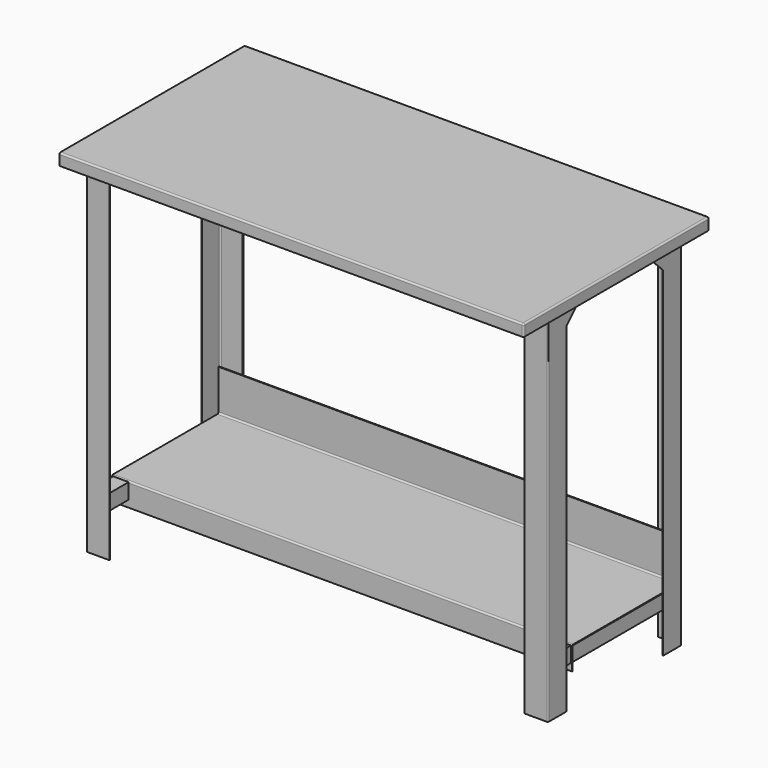
from build123d import *

# Parameters (mm, degrees)
F0_W          = 1524
F0_H          = 762
F1_DEPTH      = 2.65684
F2_W          = 2.65684
F2_H          = 2.65684
F2_W_2        = 1518.68632
F2_H_2        = 756.68632
F3_DEPTH      = 38.1
F4_R          = 5.31368
F6_DEPTH      = 1193.8
F7_R          = 3.98526
F8_R          = 3.98526
F9_W          = 50.8
F9_H          = 50.8
F10_DEPTH     = 542.85896
F12_DEPTH     = 1508.05896
F13_T1_DEPTH  = 1423.88844
F13_T6_DEPTH  = 1533.45896
F13_T9_DEPTH  = 1398.48844
F13_T14_DEPTH = 1533.45896
F13_T19_DEPTH = 1533.45896
F13_T24_DEPTH = 1533.45896
F13_T30_DEPTH = 1533.45896
F15_DEPTH     = 2.65684
F17_DEPTH     = 2.65684
F19_DEPTH     = 2.65684


# Not quite as in the source:
# - a fillet or chamfer that OpenCascade refuses, or shapes differently, is made with other operations: its cross-section is extruded or revolved along the edge and cut away or added
# - a pattern or mirror of a feature is missing from the dataset's text; its kind, count and spacing are read off the source's solid


with BuildPart() as f1:
    # F0 (on Top) → F1 (new body)
    with BuildSketch(Plane.XY):
        Rectangle(F0_W, F0_H)
    extrude(amount=F1_DEPTH)

    # F2 (on face) → F3 (join)
    with BuildSketch(Plane.XY.offset(2.65684)):
        with Locations((-760.67158, -379.67158)):
            Rectangle(F2_W, F2_H)
        with Locations((0, -379.67158)):
            Rectangle(F2_W_2, F2_H)
        with Locations((-760.67158, 0)):
            Rectangle(F2_W, F2_H_2)
        with Locations((760.67158, -379.67158)):
            Rectangle(F2_W, F2_H)
        with Locations((-760.67158, 379.67158)):
            Rectangle(F2_W, F2_H)
        with Locations((760.67158, 0)):
            Rectangle(F2_W, F2_H_2)
        with Locations((0, 379.67158)):
            Rectangle(F2_W_2, F2_H)
        with Locations((760.67158, 379.67158)):
            Rectangle(F2_W, F2_H)
    extrude(amount=-F3_DEPTH)

    # F4
    f4_edges = [f1.edges().sort_by_distance(p)[0] for p in [
        (-762, -381, -16.39316),
        (762, -381, -16.39316),
        (762, 381, -16.39316),
        (-762, 381, -16.39316),
        (-762, 0, 2.65684),
        (0, 381, 2.65684),
        (0, -381, 2.65684),
        (762, 0, 2.65684),
    ]]
    fillet(f4_edges, radius=F4_R)

    # F5 (on face) → F6 (join)
    with BuildSketch(Plane.XY.offset(2.65684)):
        Polygon((-680.48632, 274.08632), (-756.68632, 274.08632), (-756.68632, 197.88632), (-754.02948, 197.88632), (-754.02948, 271.42948), (-680.48632, 271.42948), align=None)
        Polygon((754.02948, 197.88632), (756.68632, 197.88632), (756.68632, 274.08632), (680.48632, 274.08632), (680.48632, 271.42948), (754.02948, 271.42948), align=None)
        Polygon((680.48632, -271.42948), (680.48632, -274.08632), (756.68632, -274.08632), (756.68632, -197.88632), (754.02948, -197.88632), (754.02948, -271.42948), align=None)
        Polygon((-754.02948, -197.88632), (-756.68632, -197.88632), (-756.68632, -274.08632), (-680.48632, -274.08632), (-680.48632, -271.42948), (-754.02948, -271.42948), align=None)
    extrude(amount=-F6_DEPTH)

    # F7
    f7_edges = [f1.edges().sort_by_distance(p)[0] for p in [
        (756.68632, 274.08632, -595.57158),
        (-756.68632, 274.08632, -595.57158),
        (-756.68632, -274.08632, -595.57158),
        (756.68632, -274.08632, -595.57158),
    ]]
    fillet(f7_edges, radius=F7_R)

    # F8
    f8_edges = [f1.edges().sort_by_distance(p)[0] for p in [
        (-754.02948, -271.42948, -595.57158),
        (-754.02948, 271.42948, -595.57158),
        (754.02948, -271.42948, -595.57158),
        (754.02948, 271.42948, -595.57158),
    ]]
    fillet(f8_edges, radius=F8_R)

    # F9 (on face) → F10 (join, through all)
    with BuildSketch(Plane(origin=(0, -271.42948, 0), x_dir=(-1, 0, 0), z_dir=(0, 1, 0))):
        with Locations((724.64422, -1038.74316)):
            Rectangle(F9_W, F9_H)
        with Locations((-724.64422, -1038.74316)):
            Rectangle(F9_W, F9_H)
    extrude(amount=F10_DEPTH)

    # F11 (on face) → F12 (join, through all)
    with BuildSketch(Plane(origin=(754.02948, 0, 0), x_dir=(0, -1, 0), z_dir=(-1, 0, 0))):
        Polygon((-267.44422, -876.0097688131), (-267.44422, -1013.34316), (169.82948, -1013.34316), (169.82948, -1086.88632), (172.48632, -1086.88632), (172.48632, -1010.68632), (-264.78738, -1010.68632), (-264.78738, -876.0097688131), align=None)
    extrude(amount=F12_DEPTH)

    # F13: fillet of radius 5.08 on 4 edges, made by hand

    # F13_s2 → F13_t1 (join)
    with BuildSketch(Plane.YZ.offset(-711.94422)):
        with BuildLine():
            ThreePointArc((-169.82948, -1018.42316), (-168.3415824484, -1014.8310575516), (-164.74948, -1013.34316))
            Line((-164.74948, -1013.34316), (-169.82948, -1013.34316))
            Line((-169.82948, -1013.34316), (-169.82948, -1018.42316))
        make_face()
    extrude(amount=F13_T1_DEPTH)


with BuildPart() as f13_tool4:
    # F13_s5 → F13_t6 (new body)
    with BuildSketch(Plane.YZ.offset(766.72948)):
        with BuildLine():
            ThreePointArc((264.78738, -1005.60632), (263.2994824484, -1009.1984224484), (259.70738, -1010.68632))
            Line((259.70738, -1010.68632), (264.78738, -1010.68632))
            Line((264.78738, -1010.68632), (264.78738, -1005.60632))
        make_face()
    extrude(amount=-F13_T6_DEPTH)

    split(bisect_by=Plane.YZ.offset(-756.68632), keep=Keep.TOP)

    split(bisect_by=Plane.YZ.offset(756.68632), keep=Keep.BOTTOM)


with BuildPart() as f1_1:
    add(f1.part)

    # F13_t3: union F13_tool4
    add(f13_tool4.part)

    # F13_s10 → F13_t9 (cut)
    with BuildSketch(Plane.YZ.offset(-699.24422)):
        with BuildLine():
            ThreePointArc((267.44422, -1008.26316), (265.9563224484, -1011.8552624484), (262.36422, -1013.34316))
            Line((262.36422, -1013.34316), (267.44422, -1013.34316))
            Line((267.44422, -1013.34316), (267.44422, -1008.26316))
        make_face()
    extrude(amount=F13_T9_DEPTH, mode=Mode.SUBTRACT)


with BuildPart() as f13_tool12:
    # F13_s13 → F13_t14 (new body)
    with BuildSketch(Plane.YZ.offset(766.72948)):
        with BuildLine():
            ThreePointArc((-167.40632, -1010.68632), (-170.9984224484, -1012.1742175516), (-172.48632, -1015.76632))
            Line((-172.48632, -1015.76632), (-172.48632, -1010.68632))
            Line((-172.48632, -1010.68632), (-167.40632, -1010.68632))
        make_face()
    extrude(amount=-F13_T14_DEPTH)

    split(bisect_by=Plane.XY.offset(-1013.34316), keep=Keep.TOP)


with BuildPart() as f1_2:
    add(f1_1.part)

    # F13_t11: cut F13_tool12
    add(f13_tool12.part, mode=Mode.SUBTRACT)


with BuildPart() as f13_tool17:
    # F13_s18 → F13_t19 (new body)
    with BuildSketch(Plane.YZ.offset(766.72948)):
        with BuildLine():
            ThreePointArc((-167.40632, -1010.68632), (-170.9984224484, -1012.1742175516), (-172.48632, -1015.76632))
            Line((-172.48632, -1015.76632), (-172.48632, -1010.68632))
            Line((-172.48632, -1010.68632), (-167.40632, -1010.68632))
        make_face()
    extrude(amount=-F13_T19_DEPTH)

    split(bisect_by=Plane.YZ.offset(750.04422), keep=Keep.TOP)


with BuildPart() as f1_3:
    add(f1_2.part)

    # F13_t16: cut F13_tool17
    add(f13_tool17.part, mode=Mode.SUBTRACT)


with BuildPart() as f13_tool22:
    # F13_s23 → F13_t24 (new body)
    with BuildSketch(Plane.YZ.offset(766.72948)):
        with BuildLine():
            ThreePointArc((-167.40632, -1010.68632), (-170.9984224484, -1012.1742175516), (-172.48632, -1015.76632))
            Line((-172.48632, -1015.76632), (-172.48632, -1010.68632))
            Line((-172.48632, -1010.68632), (-167.40632, -1010.68632))
        make_face()
    extrude(amount=-F13_T24_DEPTH)

    split(bisect_by=Plane.YZ.offset(-699.24422), keep=Keep.TOP)

    split(bisect_by=Plane.YZ.offset(699.24422), keep=Keep.BOTTOM)


with BuildPart() as f1_4:
    add(f1_3.part)

    # F13_t21: cut F13_tool22
    add(f13_tool22.part, mode=Mode.SUBTRACT)


with BuildPart() as f13_tool28:
    # F13_s29 → F13_t30 (new body)
    with BuildSketch(Plane.YZ.offset(766.72948)):
        with BuildLine():
            ThreePointArc((-167.40632, -1010.68632), (-170.9984224484, -1012.1742175516), (-172.48632, -1015.76632))
            Line((-172.48632, -1015.76632), (-172.48632, -1010.68632))
            Line((-172.48632, -1010.68632), (-167.40632, -1010.68632))
        make_face()
    extrude(amount=-F13_T30_DEPTH)

    split(bisect_by=Plane.YZ.offset(-750.04422), keep=Keep.BOTTOM)


with BuildPart() as f1_5:
    add(f1_4.part)

    # F13_t27: cut F13_tool28
    add(f13_tool28.part, mode=Mode.SUBTRACT)

    # F14 (on face) → F15 (join)
    with BuildSketch(Plane.XZ.offset(274.08632)):
        Polygon((-600.30106, 0), (-752.70106, 0), (-752.70106, -152.4), align=None)
        Polygon((752.70106, 0), (600.30106, 0), (752.70106, -152.4), align=None)
    f15 = extrude(amount=-F15_DEPTH)

    # F15_copies: F15 across plane
    add(f15.mirror(Plane.ZX))

    # F16 (on face) → F17 (join)
    with BuildSketch(Plane.YZ.offset(756.68632)):
        Polygon((-271.42948, -152.4), (-119.02948, 0), (-271.42948, 0), align=None)
        Polygon((119.02948, 0), (271.42948, -152.4), (271.42948, 0), align=None)
    extrude(amount=-F17_DEPTH)

    # F18 (on face) → F19 (join)
    with BuildSketch(Plane(origin=(-756.68632, 0, 0), x_dir=(0, -1, 0), z_dir=(-1, 0, 0))):
        Polygon((-271.42948, -152.4), (-119.02948, 0), (-271.42948, 0), align=None)
        Polygon((271.42948, -152.4), (271.42948, 0), (119.02948, 0), align=None)
    extrude(amount=-F19_DEPTH)


solid = f1_5.part
